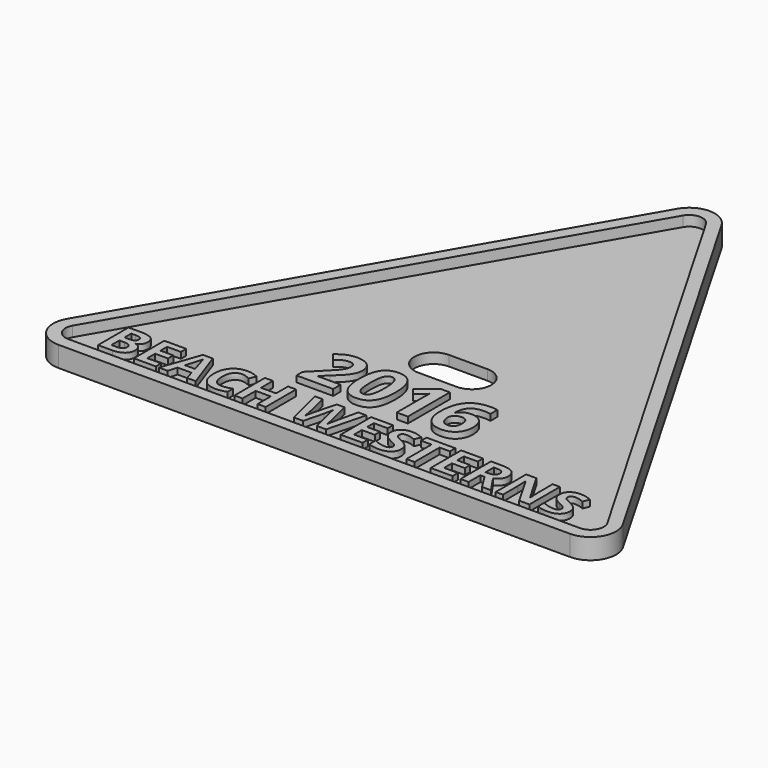
from build123d import *

# Parameters (mm, degrees)
F1_DEPTH       = 2.54
F3_DEPTH       = 2.54
F4_TEXT_SIZE   = 13.2291666667
F4_TEXT_SIZE_2 = 18.2516407222
F5_DEPTH       = 1.524


# Not quite as in the source:
# - Text() gives the source's letters only with a copy of the font that has no kerning and outlines rounded to 1/6400 em; it was checked with that copy


with BuildPart() as f1:
    # F0 (on Top) → F1 (new body)
    with BuildSketch(Plane.XY):
        with BuildLine():
            ThreePointArc((5.499261314, 76.4984841871), (0, 79.6734841871), (-5.499261314, 76.4984841871))
            Line((-5.499261314, 76.4984841871), (-68.999261314, -33.4867420935))
            ThreePointArc((-68.999261314, -33.4867420935), (-68.999261314, -39.8367420935), (-63.5, -43.0117420935))
            Line((-63.5, -43.0117420935), (63.5, -43.0117420935))
            ThreePointArc((63.5, -43.0117420935), (68.999261314, -39.8367420935), (68.999261314, -33.4867420935))
            Line((68.999261314, -33.4867420935), (5.499261314, 76.4984841871))
        make_face()
        with BuildLine():
            ThreePointArc((4.7624904754, 4.7625), (9.5248742884, 0.0346032843), (4.8316952183, -4.7619972986))
            Line((4.8316952183, -4.7619972986), (-4.7622504588, -4.7624999935))
            ThreePointArc((-4.7622504588, -4.7624999935), (-9.5249954191, 0.0066055267), (-4.7490394191, 4.7624809777))
            Line((-4.7490394191, 4.7624809777), (4.7624904754, 4.7625))
        make_face(mode=Mode.SUBTRACT)
    extrude(amount=F1_DEPTH)

    # F2 (on face) → F3 (join)
    with BuildSketch(Plane.XY.offset(2.54)):
        with BuildLine():
            Line((-5.499261314, 76.4984841871), (-68.999261314, -33.4867420935))
            ThreePointArc((-68.999261314, -33.4867420935), (-68.999261314, -39.8367420935), (-63.5, -43.0117420935))
            Line((-63.5, -43.0117420935), (63.5, -43.0117420935))
            ThreePointArc((63.5, -43.0117420935), (68.999261314, -39.8367420935), (68.999261314, -33.4867420935))
            Line((68.999261314, -33.4867420935), (5.499261314, 76.4984841871))
            ThreePointArc((5.499261314, 76.4984841871), (0, 79.6734841871), (-5.499261314, 76.4984841871))
        make_face()
        with BuildLine():
            ThreePointArc((-63.5, -39.9589209484), (-66.3554406492, -38.310331521), (-66.3554406492, -35.0131526661))
            Line((-66.3554406492, -35.0131526661), (-2.8554406492, 74.9720736145))
            ThreePointArc((-2.8554406492, 74.9720736145), (0, 76.620663042), (2.8554406492, 74.9720736145))
            Line((2.8554406492, 74.9720736145), (66.3554406492, -35.0131526661))
            ThreePointArc((66.3554406492, -35.0131526661), (66.3554406492, -38.310331521), (63.5, -39.9589209484))
            Line((63.5, -39.9589209484), (-63.5, -39.9589209484))
        make_face(mode=Mode.SUBTRACT)
    extrude(amount=F3_DEPTH)

    # F4 (on face) → F5 (join)
    with BuildSketch(Plane.XY.offset(2.54)):
        with Locations((-59.8135332834, -36.7893784839)):
            Text('BEACH WESTERNS', F4_TEXT_SIZE, font='Open Sans', font_style=FontStyle.BOLD, text_align=(TextAlign.LEFT, TextAlign.BOTTOM))
        with Locations((-21.3691485114, -22.7105477825)):
            Text('2016', F4_TEXT_SIZE_2, font='Open Sans', font_style=FontStyle.BOLD, text_align=(TextAlign.LEFT, TextAlign.BOTTOM))
    extrude(amount=F5_DEPTH)


solid = f1.part
